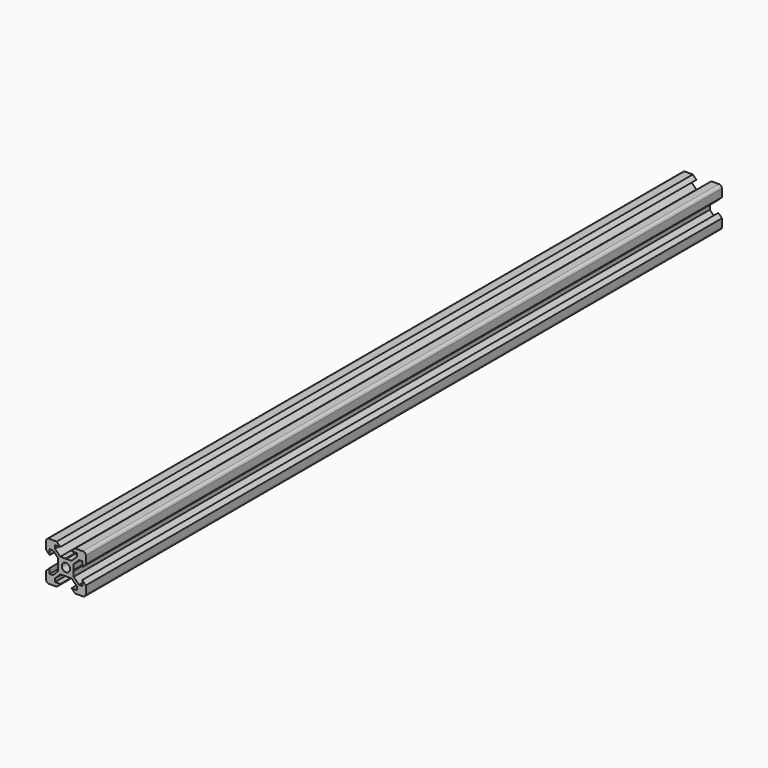
from build123d import *

# Parameters (mm, degrees)
F0_R     = 2.1
F1_DEPTH = 200


# Not quite as in the source:
# - ends of sketch curves that miss each other by under 0.0002 mm in the source are joined


with BuildPart() as f1:
    # F0 (on Front) → F1 (new body, symmetric)
    with BuildSketch(Plane.XZ):
        with BuildLine():
            Line((-4.64, 10.000002), (-8.500001, 10.000002))
            ThreePointArc((-8.500001, 10.000002), (-9.5606615253, 9.5606618182), (-10.000001, 8.500001))
            Line((-10.000001, 8.500001), (-10.000001, 4.640001))
            Line((-10.000001, 4.640001), (-8.199999, 2.840001))
            Line((-8.199999, 2.840001), (-8.199999, 5.499339))
            Line((-8.199999, 5.499339), (-6.56, 5.499339))
            Line((-6.56, 5.499339), (-3.90066, 2.840001))
            Line((-3.90066, 2.840001), (-3.90066, 0.2))
            Line((-3.90066, 0.2), (-3.70066, 0))
            Line((-3.70066, 0), (-3.90066, -0.2))
            Line((-3.90066, -0.2), (-3.90066, -2.840001))
            Line((-3.90066, -2.840001), (-6.56, -5.499341))
            Line((-6.56, -5.499341), (-8.199999, -5.499341))
            Line((-8.199999, -5.499341), (-8.199999, -2.840001))
            Line((-8.199999, -2.840001), (-10.000001, -4.640001))
            Line((-10.000001, -4.640001), (-10.000001, -8.500001))
            ThreePointArc((-10.000001, -8.500001), (-9.5606608182, -9.5606615253), (-8.500001, -10.000001))
            Line((-8.500001, -10.000001), (-4.64, -10.000001))
            Line((-4.64, -10.000001), (-2.84, -8.2))
            Line((-2.84, -8.2), (-5.49934, -8.2))
            Line((-5.49934, -8.2), (-5.49934, -6.560001))
            Line((-5.49934, -6.560001), (-2.84, -3.900661))
            Line((-2.84, -3.900661), (-0.199999, -3.900661))
            Line((-0.199999, -3.900661), (1e-06, -3.700661))
            Line((1e-06, -3.700661), (0.200001, -3.900661))
            Line((0.200001, -3.900661), (2.84, -3.900661))
            Line((2.84, -3.900661), (5.499342, -6.560001))
            Line((5.499342, -6.560001), (5.499342, -8.2))
            Line((5.499342, -8.2), (2.84, -8.2))
            Line((2.84, -8.2), (4.64, -10.000001))
            Line((4.64, -10.000001), (8.500001, -10.000001))
            ThreePointArc((8.500001, -10.000001), (9.5606611718, -9.5606611718), (10.000001, -8.500001))
            Line((10.000001, -8.500001), (10.000001, -4.640001))
            Line((10.000001, -4.640001), (8.200001, -2.840001))
            Line((8.200001, -2.840001), (8.200001, -5.499341))
            Line((8.200001, -5.499341), (6.560002, -5.499341))
            Line((6.560002, -5.499341), (3.90066, -2.840001))
            Line((3.90066, -2.840001), (3.90066, -0.2))
            Line((3.90066, -0.2), (3.70066, 0))
            Line((3.70066, 0), (3.90066, 0.2))
            Line((3.90066, 0.2), (3.90066, 2.840001))
            Line((3.90066, 2.840001), (6.560002, 5.499339))
            Line((6.560002, 5.499339), (8.200001, 5.499339))
            Line((8.200001, 5.499339), (8.200001, 2.840001))
            Line((8.200001, 2.840001), (10.000001, 4.640001))
            Line((10.000001, 4.640001), (10.000001, 8.500002))
            ThreePointArc((10.000001, 8.500002), (9.5606611718, 9.5606621718), (8.500001, 10.000002))
            Line((8.500001, 10.000002), (4.64, 10.000002))
            Line((4.64, 10.000002), (2.84, 8.200002))
            Line((2.84, 8.200002), (5.499342, 8.200002))
            Line((5.499342, 8.200002), (5.499342, 6.559999))
            Line((5.499342, 6.559999), (2.84, 3.900661))
            Line((2.84, 3.900661), (0.200001, 3.900661))
            Line((0.200001, 3.900661), (1e-06, 3.700661))
            Line((1e-06, 3.700661), (-0.199999, 3.900661))
            Line((-0.199999, 3.900661), (-2.84, 3.900661))
            Line((-2.84, 3.900661), (-5.49934, 6.559999))
            Line((-5.49934, 6.559999), (-5.49934, 8.200002))
            Line((-5.49934, 8.200002), (-2.84, 8.200002))
            Line((-2.84, 8.200002), (-4.64, 10.000002))
        make_face()
        with Locations((1e-06, 0)):
            Circle(F0_R, mode=Mode.SUBTRACT)
    extrude(amount=F1_DEPTH, both=True)


with BuildPart() as f1_1:
    # F2: moved
    add(f1.part.moved(Location((0, 200, 0))))


solid = f1_1.part
